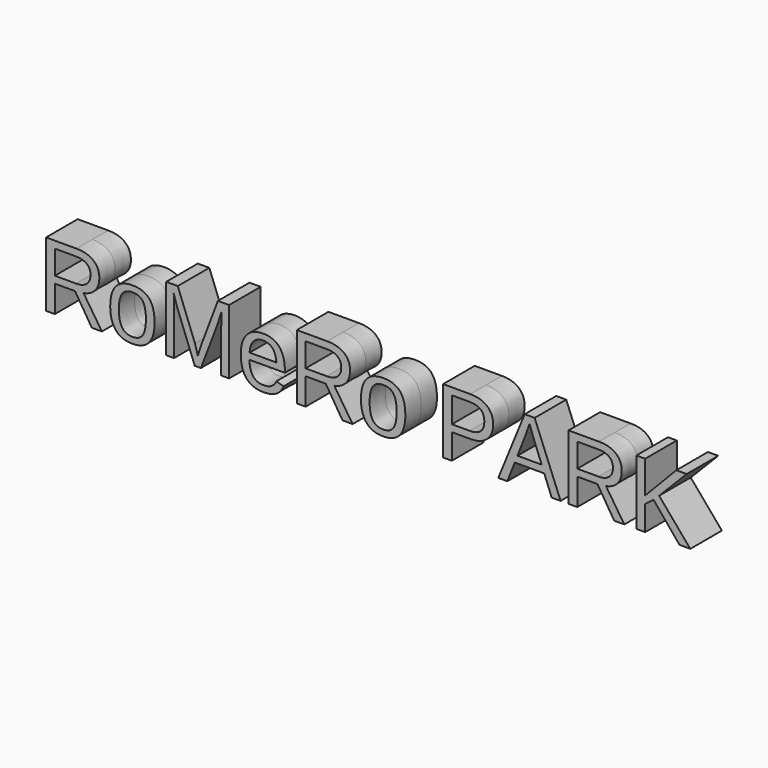
from build123d import *

# Parameters (mm, degrees)
F0_TEXT_SIZE = 60.4634483655
F1_DEPTH     = 12.7


# Not quite as in the source:
# - the program builds the solid bodies; features that only make, move or delete a surface that nothing else refers to are left out
# - Text() gives the source's letters only with a copy of the font that has no kerning and outlines rounded to 1/6400 em; it was checked with that copy


with BuildPart() as f1:
    # F0 (on Front) → F1 (new body, symmetric)
    with BuildSketch(Plane.XZ):
        with Locations((-211.7685041934, 0)):
            Text('RoMeRo PARK', F0_TEXT_SIZE, font='Arimo', text_align=(TextAlign.LEFT, TextAlign.BOTTOM))
    extrude(amount=F1_DEPTH, both=True)


solid = f1.part
